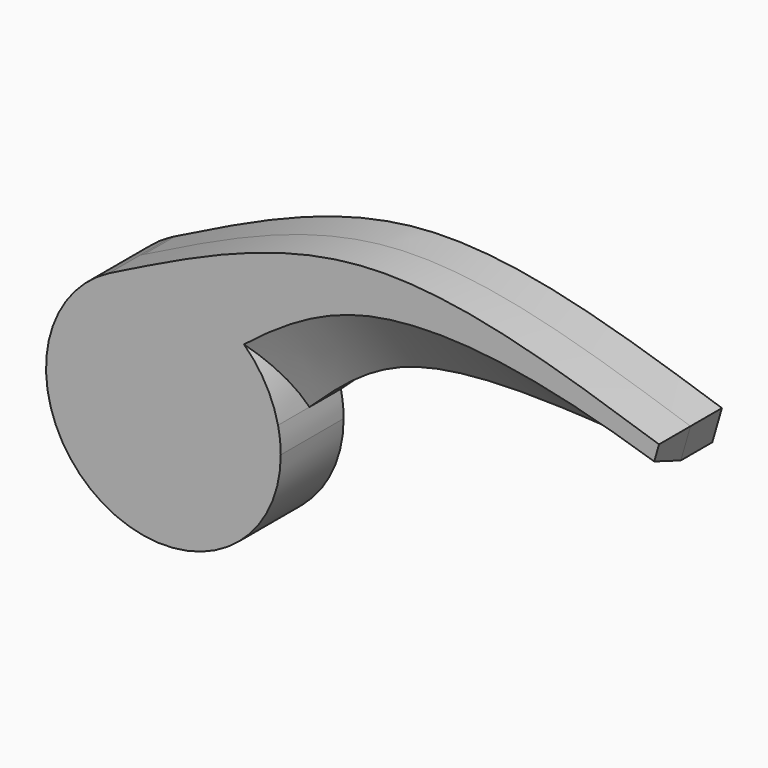
from build123d import *

# Parameters (mm, degrees)
F6_DEPTH = 10
F7_DEPTH = 20


# Not quite as in the source:
# - the dataset's text gives a spline's control points without its knots; the knots are read off the source's solid


with BuildPart() as f5:
    # F3 (on offset) → F5 section 0
    with BuildSketch(Plane.XZ.offset(10)):
        with BuildLine():
            ThreePointArc((-75.5787535417, 16.7525420321), (-74.2842309522, -36.7668523877), (-32.5165676908, -3.2785906609))
            add(Edge.make_bspline(
                [(-32.5165676908, -3.2785906609), (-25.0186225888, 3.7525831829), (-6.6027990329, 21.0474968683), (36.4369216658, 17.5617465832), (61.9822815061, 15.4927987605)],
                knots=[0, 0, 0, 0, 0.406452044, 1, 1, 1, 1], degree=3))
            Line((61.9822815061, 15.4927987605), (64.4333958626, 23.9602774382))
            add(Edge.make_bspline(
                [(-75.5787535417, 16.7525420321), (-54.628951456, 27.285399841), (-11.406645731, 48.9685404457), (38.647869417, 32.4670255034), (64.4333958626, 23.9602774382)],
                knots=[0, 0, 0, 0, 0.4849009259, 1, 1, 1, 1], degree=3))
        make_face()
    # F4 (on offset) → F5 section 1
    with BuildSketch(Plane.XZ.offset(20)):
        with BuildLine():
            add(Edge.make_bspline(
                [(-75.5787535417, 16.7525420321), (-54.628951456, 27.285399841), (-11.406645731, 48.9685404457), (38.647869417, 32.4670255034), (64.4333958626, 23.9602774382)],
                knots=[0, 0, 0, 0, 0.4849009259, 1, 1, 1, 1], degree=3))
            ThreePointArc((-75.5787535417, 16.7525420321), (-65.7534042192, -39.2752402765), (-41.1793711539, 12.0255080478))
            add(Edge.make_bspline(
                [(-41.1793711539, 12.0255080478), (-25.2502910967, 24.6854926251), (-0.0760708598, 33.9443363857), (36.1576432322, 28.3926800744), (63.2078386843, 19.7265380993)],
                knots=[0, 0, 0, 0, 0.4558632428, 1, 1, 1, 1], degree=3))
            Line((63.2078386843, 19.7265380993), (64.4333958626, 23.9602774382))
        make_face()
    loft()

    # F0 (on Front) → F6 (join)
    with BuildSketch(Plane.XZ):
        with BuildLine():
            ThreePointArc((-74.6210650057, 17.2339850929), (-48.6067992872, 17.1628264037), (-32.5165676908, -3.2785906609))
            add(Edge.make_bspline(
                [(-32.5165676908, -3.2785906609), (-25.0186225888, 3.7525831829), (-6.6027990329, 21.0474968683), (36.4369216658, 17.5617465832), (61.9822815061, 15.4927987605)],
                knots=[0, 0, 0, 0, 0.406452044, 1, 1, 1, 1], degree=3))
            Line((61.9822815061, 15.4927987605), (64.4333958626, 23.9602774382))
            add(Edge.make_bspline(
                [(-74.6210650057, 17.2339850929), (-53.9898610909, 27.6037376874), (-11.0368055784, 48.8466149254), (38.647869417, 32.4670255034), (64.4333958626, 23.9602774382)],
                knots=[0.0073887471, 0.0073887471, 0.0073887471, 0.0073887471, 0.4849009259, 1, 1, 1, 1], degree=3))
        make_face()
    extrude(amount=F6_DEPTH)

    # F0 (on Front) → F7 (join)
    with BuildSketch(Plane.XZ):
        with BuildLine():
            ThreePointArc((-75.5787535417, 16.7525420321), (-77.1329137918, -35.2493874652), (-31.8209869176, -9.6868099645))
            ThreePointArc((-31.8209869176, -9.6868099645), (-31.9953913254, -6.4638801151), (-32.5165676908, -3.2785906609))
            ThreePointArc((-32.5165676908, -3.2785906609), (-48.6067992872, 17.1628264037), (-74.6210650057, 17.2339850929))
            add(Edge.make_bspline(
                [(-75.5787535417, 16.7525420321), (-75.2595279418, 16.9130379566), (-74.940300314, 17.0735295431), (-74.6210650057, 17.2339850929)],
                knots=[0, 0, 0, 0, 0.0073887471, 0.0073887471, 0.0073887471, 0.0073887471], degree=3))
        make_face()
    extrude(amount=F7_DEPTH)


solid = f5.part
